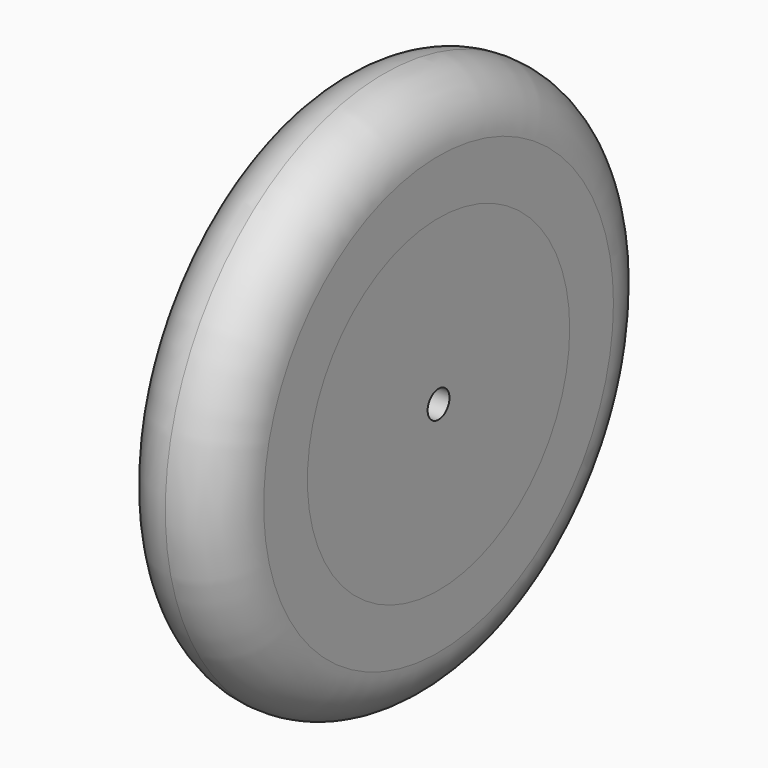
from build123d import *

# Parameters (mm, degrees)
F0_R     = 19.05
F0_R_2   = 1.5875
F1_DEPTH = 6.35
F0_R_3   = 31.75
F2_DEPTH = 6.35
F3_R     = 6.34999


# Not quite as in the source:
# - a fillet or chamfer is up to 0.001 mm smaller than in the source, because OpenCascade refuses the exact size


with BuildPart() as f1:
    # F0 (on Right) → F1 (new body, symmetric)
    with BuildSketch(Plane.YZ):
        Circle(F0_R)
        Circle(F0_R_2, mode=Mode.SUBTRACT)
    extrude(amount=F1_DEPTH, both=True)


with BuildPart() as f2:
    # F0 (on Right) → F2 (new body, symmetric)
    with BuildSketch(Plane.YZ):
        Circle(F0_R_3)
        Circle(F0_R, mode=Mode.SUBTRACT)
    extrude(amount=F2_DEPTH, both=True)

    # F3 (radius 6.35 in the source; OpenCascade refuses exactly that, so slightly less here)
    f3_edges = [f2.edges().sort_by_distance(p)[0] for p in [
        (6.35, -31.75, 0),
        (-6.35, -31.75, 0),
    ]]
    fillet(f3_edges, radius=F3_R)


solid = Compound([f1.part, f2.part])
